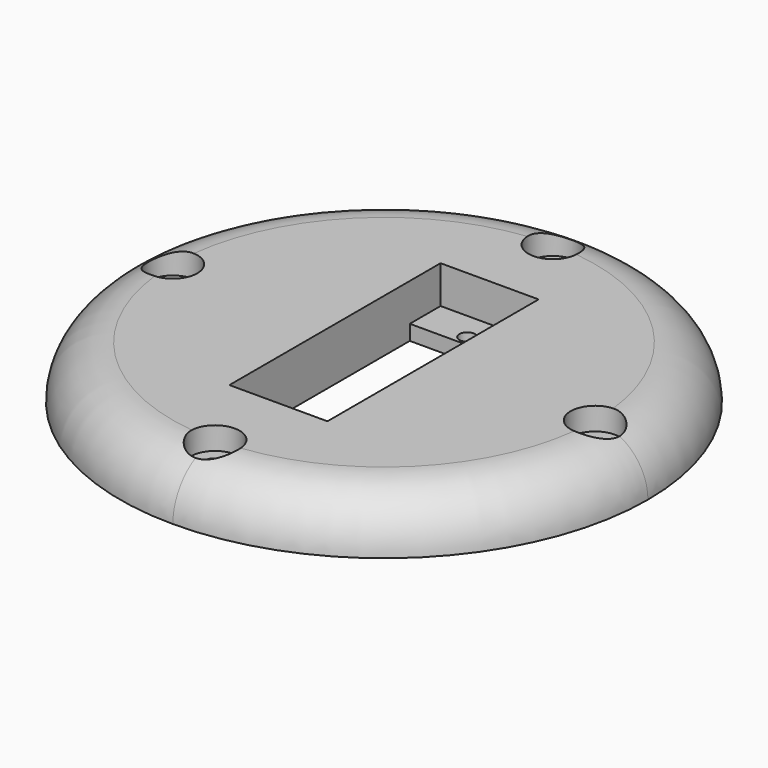
from build123d import *

# Parameters (mm, degrees)
F0_W          = 70
F0_H          = 70
F1_DEPTH      = 10
F2_W          = 13
F2_H          = 24.8
F3_DEPTH      = 25
F4_W          = 70
F4_H          = 70
F4_W_2        = 40
F4_H_2        = 40
F5_DEPTH      = 4
F6_W          = 13
F6_H          = 35
F7_DEPTH      = 9
F8_R          = 1.05
F9_DEPTH      = 25
F10_R         = 1.6
F11_DEPTH     = 25
F12_R         = 3.25
F13_DEPTH     = 3
F14_DEPTH     = 4
F15_R         = 34.99999
F16_DEPTH     = 1
F17_T1_DEPTH  = 2e-05
F17_T3_DEPTH  = 2e-05
F17_T6_ANGLE  = 90
F17_T8_ANGLE  = 90
F17_T10_ANGLE = 90
F17_T12_ANGLE = 90


# Not quite as in the source:
# - a fillet or chamfer that OpenCascade refuses, or shapes differently, is made with other operations: its cross-section is extruded or revolved along the edge and cut away or added
# - a fillet or chamfer is up to 0.001 mm smaller than in the source, because OpenCascade refuses the exact size


with BuildPart() as f1:
    # F0 (on Top) → F1 (new body)
    with BuildSketch(Plane.XY):
        Rectangle(F0_W, F0_H)
    extrude(amount=F1_DEPTH)

    # F2 (on face) → F3 (cut)
    with BuildSketch(Plane.XY.offset(10)):
        Rectangle(F2_W, F2_H)
    extrude(amount=-F3_DEPTH, mode=Mode.SUBTRACT)

    # F4 (on face) → F5 (cut)
    with BuildSketch(Plane.XY.offset(10)):
        Rectangle(F4_W, F4_H)
        Rectangle(F4_W_2, F4_H_2, mode=Mode.SUBTRACT)
    extrude(amount=-F5_DEPTH, mode=Mode.SUBTRACT)

    # F6 (on face) → F7 (cut)
    with BuildSketch(Plane.XY.offset(10)):
        Rectangle(F6_W, F6_H)
    extrude(amount=-F7_DEPTH, mode=Mode.SUBTRACT)

    # F8 (on face) → F9 (cut)
    with BuildSketch(Plane.XY.offset(1)):
        with Locations((0, 13.8)):
            Circle(F8_R)
        with Locations((0, -13.8)):
            Circle(F8_R)
    extrude(amount=-F9_DEPTH, mode=Mode.SUBTRACT)

    # F10 (on face) → F11 (cut)
    with BuildSketch(Plane.XY.offset(6)):
        with Locations((-28, 0)):
            Circle(F10_R)
        with Locations((28, 0)):
            Circle(F10_R)
        with Locations((0, -28)):
            Circle(F10_R)
        with Locations((0, 28)):
            Circle(F10_R)
    extrude(amount=-F11_DEPTH, mode=Mode.SUBTRACT)

    # F12 (on face) → F13 (cut)
    with BuildSketch(Plane.XY.offset(6)):
        with Locations((-28, 0)):
            Circle(F12_R)
        with Locations((28, 0)):
            Circle(F12_R)
        with Locations((0, -28)):
            Circle(F12_R)
        with Locations((0, 28)):
            Circle(F12_R)
    extrude(amount=-F13_DEPTH, mode=Mode.SUBTRACT)

    # F14 (cut, through all): a face of the model
    f14_faces = [f1.faces().sort_by_distance(p)[0] for p in [
        (-19.4343145751, 0, 10),
    ]]
    extrude(f14_faces, amount=-F14_DEPTH, mode=Mode.SUBTRACT)

    # F15 (radius 35 in the source; OpenCascade refuses exactly that, so slightly less here)
    f15_edges = [f1.edges().sort_by_distance(p)[0] for p in [
        (-35, -35, 3),
        (35, -35, 3),
        (35, 35, 3),
        (-35, 35, 3),
    ]]
    fillet(f15_edges, radius=F15_R)

    # F16 (add): a face of the model
    f16_faces = [f1.faces().sort_by_distance(p)[0] for p in [
        (0, -34.0100505063, 0),
    ]]
    extrude(f16_faces, amount=F16_DEPTH)

    # F17: fillet of radius 7 on 1 edges, made by hand

    # F17_s2 → F17_t1 (cut)
    with BuildSketch(Plane.YZ.offset(-1e-05)):
        with BuildLine():
            ThreePointArc((-35, -1), (-32.9497474683, 3.9497474683), (-28, 6))
            Line((-28, 6), (-35, 6))
            Line((-35, 6), (-35, -1))
        make_face()
        with BuildLine():
            ThreePointArc((35, -1), (32.9497474683, 3.9497474683), (28, 6))
            Line((28, 6), (35, 6))
            Line((35, 6), (35, -1))
        make_face()
    extrude(amount=F17_T1_DEPTH, mode=Mode.SUBTRACT)

    # F17_s4 → F17_t3 (cut)
    with BuildSketch(Plane.XZ.offset(-1e-05)):
        with BuildLine():
            ThreePointArc((35, -1), (32.9497474683, 3.9497474683), (28, 6))
            Line((28, 6), (35, 6))
            Line((35, 6), (35, -1))
        make_face()
        with BuildLine():
            ThreePointArc((-35, -1), (-32.9497474683, 3.9497474683), (-28, 6))
            Line((-28, 6), (-35, 6))
            Line((-35, 6), (-35, -1))
        make_face()
    extrude(amount=F17_T3_DEPTH, mode=Mode.SUBTRACT)

    # F17_s5 → F17_t6 (revolve, cut)
    with BuildSketch(Plane.YZ.offset(1e-05)):
        with BuildLine():
            ThreePointArc((-35, -1), (-32.9497474683, 3.9497474683), (-28, 6))
            Line((-28, 6), (-35, 6))
            Line((-35, 6), (-35, -1))
        make_face()
    revolve(axis=Axis((1e-05, -1e-05, 6), (0, 0, 1)), revolution_arc=F17_T6_ANGLE, mode=Mode.SUBTRACT)

    # F17_s7 → F17_t8 (revolve, cut)
    with BuildSketch(Plane.XZ.offset(-1e-05)):
        with BuildLine():
            ThreePointArc((35, -1), (32.9497474683, 3.9497474683), (28, 6))
            Line((28, 6), (35, 6))
            Line((35, 6), (35, -1))
        make_face()
    revolve(axis=Axis((1e-05, 1e-05, 6), (0, 0, 1)), revolution_arc=F17_T8_ANGLE, mode=Mode.SUBTRACT)

    # F17_s9 → F17_t10 (revolve, cut)
    with BuildSketch(Plane.XZ.offset(-1e-05)):
        with BuildLine():
            ThreePointArc((-35, -1), (-32.9497474683, 3.9497474683), (-28, 6))
            Line((-28, 6), (-35, 6))
            Line((-35, 6), (-35, -1))
        make_face()
    revolve(axis=Axis((-1e-05, 1e-05, 6), (0, 0, -1)), revolution_arc=F17_T10_ANGLE, mode=Mode.SUBTRACT)

    # F17_s11 → F17_t12 (revolve, cut)
    with BuildSketch(Plane.YZ.offset(-1e-05)):
        with BuildLine():
            ThreePointArc((-28, 6), (-32.9497474683, 3.9497474683), (-35, -1))
            Line((-35, -1), (-35, 6))
            Line((-35, 6), (-28, 6))
        make_face()
    revolve(axis=Axis((-1e-05, -1e-05, 6), (0, 0, -1)), revolution_arc=F17_T12_ANGLE, mode=Mode.SUBTRACT)


solid = f1.part
